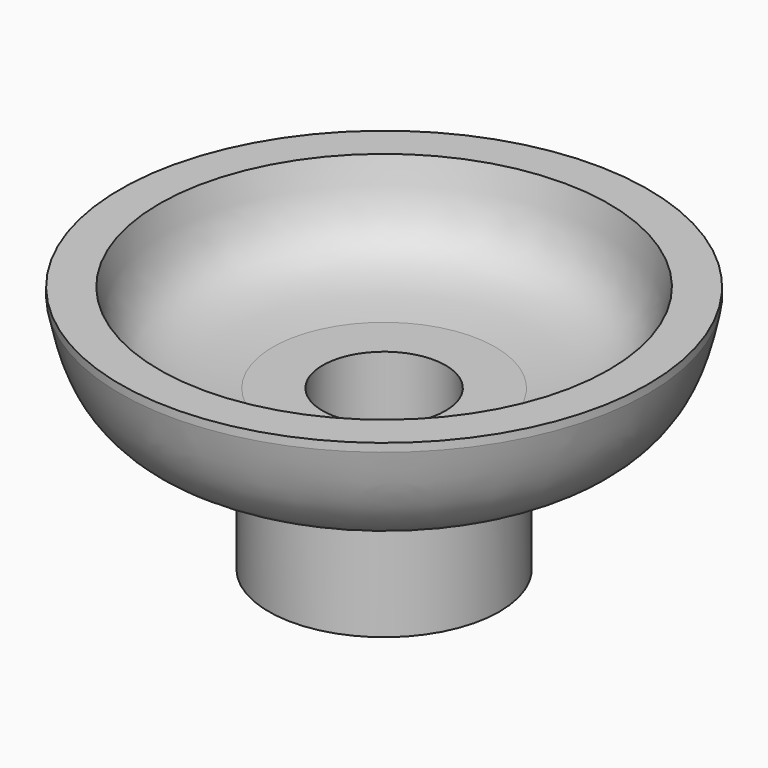
from build123d import *


# Not quite as in the source:
# - the dataset's text gives a spline's control points without its knots; the knots are read off the source's solid


with BuildPart() as f1:
    # F0 (on Front) → F1 (revolve)
    with BuildSketch(Plane.XZ):
        with BuildLine():
            Line((59.1187243464, 34.4952046871), (43.9585000277, 34.4952046871))
            add(Edge.make_bspline(
                [(43.9585000277, 34.4952046871), (41.8918768311, 24.700407418), (37.5100254604, 3.932545182), (12.96748339, 1.3595089234), (0, 0)],
                knots=[0, 0, 0, 0, 0.471632427, 1, 1, 1, 1], degree=3))
            Line((0, 0), (-19.2318391055, 0))
            Line((-19.2318391055, 0), (-19.2318391055, -61.6640076041))
            Line((-19.2318391055, -61.6640076041), (1.6155341416, -61.6640076041))
            Line((1.6155341416, -61.6640076041), (1.6155341416, -15.4095436873))
            add(Edge.make_bspline(
                [(59.1187243464, 31.2965196729), (58.8448586357, 29.9985282832), (58.2781105276, 27.3103366025), (57.2988143451, 23.050693641), (56.0968982517, 18.599669286), (54.5509849079, 13.9859685976), (52.8439715575, 10.0349429883), (51.1284333409, 6.8509402442), (49.6402745205, 4.4706401265), (47.9262273076, 2.1237916395), (46.2933009209, 0.2248578691), (44.8593170754, -1.2389494825), (43.9099024438, -2.1260156961), (43.1189162519, -2.8157853262), (42.3204145906, -3.4809169859), (41.3063811118, -4.2701681718), (40.0705820175, -5.1510468779), (38.4033145852, -6.2415778101), (35.4482818213, -7.9406844275), (31.1828714875, -9.843185835), (26.0855859435, -11.5102722871), (21.0330221915, -12.7372398848), (16.0357539234, -13.6532824792), (11.1089724523, -14.3555620415), (6.2791061999, -14.9208035067), (3.149443021, -15.2487289211), (1.6155341416, -15.4095436873)],
                knots=[1e-10, 1e-10, 1e-10, 1e-10, 0.0625000001, 0.1250000001, 0.1875000001, 0.2500000001, 0.3125000001, 0.3437500001, 0.3750000001, 0.4062500001, 0.4375000001, 0.4531250001, 0.4687500001, 0.4765625001, 0.4843750001, 0.5000000001, 0.5156250001, 0.5312500001, 0.5625, 0.625, 0.6875, 0.75, 0.8125, 0.875, 0.9375, 1, 1, 1, 1], degree=3))
            Line((59.1187243464, 31.2965196729), (59.1187243464, 34.4952046871))
        make_face()
    revolve(axis=Axis((-43.0426932871, 0, -13.5844014585), (0, 0, -1)))


solid = f1.part
